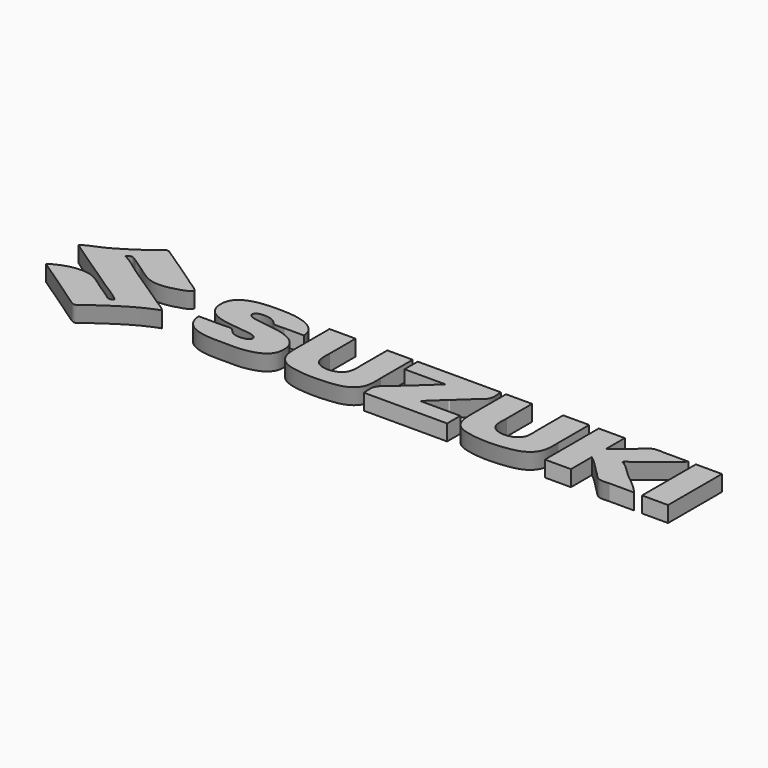
from build123d import *

# Parameters (mm, degrees)
F1_DEPTH = 25
F0_W     = 41
F0_H     = 106


# Not quite as in the source:
# - ends of sketch curves that miss each other by under 0.0002 mm in the source are joined


with BuildPart() as f1:
    # F0 (on Top) → F1 (new body)
    with BuildSketch(Plane.XY):
        Polygon((-498.7323, 35.60855), (-499.5, 35.04365), (-498.6864, 34.46155), (-497.8721, 33.88035), (-497.0571, 33.30005), (-496.2415, 32.72065), (-495.4252, 32.14205), (-494.6084, 31.56425), (-493.7909, 30.98735), (-492.9728, 30.41125), (-492.1542, 29.83595), (-491.335, 29.26135), (-490.5152, 28.68765), (-489.6948, 28.11455), (-488.874, 27.54235), (-488.0526, 26.97075), (-487.2306, 26.39985), (-486.4082, 25.82965), (-485.5852, 25.26015), (-484.7618, 24.69135), (-483.9379, 24.12315), (-483.1135, 23.55565), (-482.2887, 22.98865), (-481.4635, 22.42235), (-480.6378, 21.85655), (-479.8116, 21.29145), (-478.9851, 20.72675), (-478.1582, 20.16275), (-477.3309, 19.59915), (-476.5032, 19.03615), (-475.6751, 18.47365), (-474.8467, 17.91155), (-474.0179, 17.35005), (-473.1888, 16.78895), (-472.3594, 16.22825), (-471.5297, 15.66795), (-470.6997, 15.10815), (-469.8693, 14.54875), (-469.0387, 13.98965), (-468.2078, 13.43095), (-467.3767, 12.87265), (-466.5453, 12.31465), (-465.7137, 11.75695), (-464.8819, 11.19965), (-464.0498, 10.64255), (-463.2176, 10.08575), (-462.3851, 9.52925), (-461.5525, 8.97295), (-460.7197, 8.41695), (-459.8868, 7.86115), (-459.0537, 7.30555), (-458.2204, 6.75015), (-457.387, 6.19495), (-456.5536, 5.63985), (-455.72, 5.08495), (-454.8863, 4.53015), (-454.0525, 3.97545), (-453.2187, 3.42085), (-452.3848, 2.86635), (-451.5508, 2.31195), (-450.7168, 1.75765), (-449.8828, 1.20335), (-449.0488, 0.64905), (-448.2148, 0.09485), (-447.3807, -0.45945), (-446.5467, -1.01365), (-445.7127, -1.56795), (-444.8787, -2.12235), (-444.0448, -2.67665), (-443.211, -3.23115), (-442.3772, -3.78575), (-441.5435, -4.34035), (-440.7099, -4.89515), (-439.8764, -5.45005), (-439.043, -6.00505), (-438.2098, -6.56025), (-437.3766, -7.11565), (-436.5436, -7.67125), (-435.7108, -8.22695), (-434.8782, -8.78295), (-434.0457, -9.33915), (-433.2134, -9.89565), (-432.3813, -10.45245), (-431.5494, -11.00945), (-430.7178, -11.56675), (-429.8864, -12.12435), (-429.0552, -12.68225), (-428.2243, -13.24055), (-427.3936, -13.79915), (-426.5633, -14.35815), (-425.7332, -14.91745), (-424.9034, -15.47725), (-424.0739, -16.03745), (-423.2448, -16.59805), (-422.416, -17.15905), (-421.5875, -17.72055), (-420.7594, -18.28245), (-419.9316, -18.84495), (-419.1042, -19.40785), (-418.2772, -19.97135), (-417.4507, -20.53525), (-416.6245, -21.09975), (-415.7987, -21.66485), (-414.9734, -22.23055), (-414.1485, -22.79675), (-413.324, -23.36355), (-412.5, -23.93095), (-411.6765, -24.49535), (-410.8486, -25.05655), (-410.0166, -25.61485), (-409.1807, -26.17045), (-408.3413, -26.72355), (-407.4987, -27.27445), (-406.653, -27.82335), (-405.8047, -28.37065), (-404.9538, -28.91635), (-404.1008, -29.46085), (-403.2459, -30.00435), (-402.3893, -30.54705), (-401.5314, -31.08935), (-400.6724, -31.63125), (-399.8126, -32.17325), (-398.9522, -32.71535), (-398.0916, -33.25805), (-397.2309, -33.80135), (-396.3706, -34.34565), (-395.5108, -34.89105), (-394.6518, -35.43795), (-393.7939, -35.98655), (-392.9373, -36.53705), (-392.0824, -37.08975), (-391.2295, -37.64475), (-390.3787, -38.20245), (-389.5303, -38.76305), (-388.6847, -39.32685), (-387.8421, -39.89395), (-387.0028, -40.46465), (-386.167, -41.03925), (-385.3351, -41.61795), (-384.5072, -42.20105), (-383.6837, -42.78865), (-382.8649, -43.38115), (-382.0509, -43.97865), (-381.2422, -44.58155), (-380.4389, -45.19005), (-379.6413, -45.80425), (-378.8498, -46.42455), (-378.0645, -47.05115), (-377.2858, -47.68425), (-376.5139, -48.32415), (-375.7491, -48.97105), (-374.9917, -49.62525), (-374.2419, -50.28695), (-373.5, -50.95635), (-374.3581, -51.38155), (-375.2655, -51.86565), (-376.2089, -52.36255), (-377.175, -52.82615), (-378.1506, -53.21035), (-379.1225, -53.46895), (-380.0772, -53.55595), (-380.972, -53.46095), (-381.8777, -53.21815), (-382.7883, -52.85145), (-383.6974, -52.38435), (-384.5988, -51.84045), (-385.4865, -51.24355), (-386.3541, -50.61715), (-387.1955, -49.98495), (-388.0044, -49.37055), (-388.7746, -48.79765), (-389.5, -48.28975), (-409.5, -34.95635), (-410.3052, -34.41505), (-411.1114, -33.86445), (-411.9189, -33.30565), (-412.7278, -32.73955), (-413.5382, -32.16715), (-414.3504, -31.58965), (-415.1643, -31.00785), (-415.9802, -30.42275), (-416.7981, -29.83555), (-417.6183, -29.24705), (-418.4409, -28.65835), (-419.2659, -28.07045), (-420.0936, -27.48435), (-420.924, -26.90105), (-421.7574, -26.32155), (-422.5937, -25.74685), (-423.4333, -25.17805), (-424.2761, -24.61595), (-425.1225, -24.06175), (-425.9723, -23.51625), (-426.826, -22.98065), (-427.6834, -22.45595), (-428.5449, -21.94305), (-429.4105, -21.44295), (-430.2803, -20.95665), (-431.1545, -20.48535), (-432.0333, -20.02975), (-432.9168, -19.59115), (-433.805, -19.17025), (-434.6983, -18.76835), (-435.5965, -18.38625), (-436.5, -18.02505), (-437.4101, -17.68515), (-438.3275, -17.36615), (-439.252, -17.06775), (-440.1832, -16.78965), (-441.1208, -16.53165), (-442.0644, -16.29335), (-443.0137, -16.07465), (-443.9683, -15.87525), (-444.928, -15.69485), (-445.8923, -15.53315), (-446.8609, -15.38995), (-447.8336, -15.26485), (-448.8098, -15.15775), (-449.7894, -15.06825), (-450.7719, -14.99615), (-451.757, -14.94115), (-452.7445, -14.90295), (-453.7338, -14.88145), (-454.7247, -14.87615), (-455.7169, -14.88695), (-456.71, -14.91345), (-457.7037, -14.95555), (-458.6976, -15.01285), (-459.6914, -15.08505), (-460.6847, -15.17205), (-461.6772, -15.27335), (-462.6686, -15.38885), (-463.6585, -15.51825), (-464.6466, -15.66135), (-465.6325, -15.81775), (-466.6159, -15.98715), (-467.5965, -16.16945), (-468.5739, -16.36425), (-469.5478, -16.57135), (-470.5178, -16.79045), (-471.4835, -17.02125), (-472.4448, -17.26355), (-473.4011, -17.51705), (-474.3522, -17.78155), (-475.2977, -18.05665), (-476.2373, -18.34215), (-477.1706, -18.63775), (-478.0974, -18.94325), (-479.0172, -19.25825), (-479.9297, -19.58265), (-480.8346, -19.91605), (-481.7315, -20.25835), (-482.6201, -20.60905), (-483.5, -20.96795), (-484.4491, -21.36105), (-485.4051, -21.75885), (-486.3651, -22.16375), (-487.3259, -22.57815), (-488.2846, -23.00465), (-489.238, -23.44565), (-490.1831, -23.90365), (-491.1168, -24.38095), (-492.036, -24.88025), (-492.9377, -25.40375), (-493.8187, -25.95415), (-494.6761, -26.53375), (-495.5067, -27.14505), (-496.3074, -27.79045), (-497.0753, -28.47255), (-497.8072, -29.19375), (-498.5, -29.95635), (-497.6616, -30.52175), (-496.823, -31.08685), (-495.9841, -31.65165), (-495.145, -32.21625), (-494.3057, -32.78065), (-493.4661, -33.34475), (-492.6264, -33.90865), (-491.7865, -34.47245), (-490.9464, -35.03595), (-490.1061, -35.59935), (-489.2657, -36.16255), (-488.4251, -36.72555), (-487.5844, -37.28855), (-486.7436, -37.85135), (-485.9027, -38.41405), (-485.0617, -38.97665), (-484.2205, -39.53925), (-483.3793, -40.10165), (-482.5381, -40.66415), (-481.6967, -41.22645), (-480.8553, -41.78885), (-480.0139, -42.35115), (-479.1725, -42.91355), (-478.331, -43.47585), (-477.4895, -44.03825), (-476.648, -44.60065), (-475.8066, -45.16305), (-474.9651, -45.72555), (-474.1237, -46.28815), (-473.2823, -46.85085), (-472.441, -47.41355), (-471.5998, -47.97645), (-470.7586, -48.53945), (-469.9175, -49.10265), (-469.0765, -49.66595), (-468.2356, -50.22945), (-467.3949, -50.79305), (-466.5542, -51.35685), (-465.7137, -51.92095), (-464.8734, -52.48515), (-464.0332, -53.04965), (-463.1931, -53.61445), (-462.3533, -54.17935), (-461.5136, -54.74465), (-460.6742, -55.31015), (-459.8349, -55.87595), (-458.9959, -56.44215), (-458.1571, -57.00855), (-457.3185, -57.57535), (-456.4802, -58.14245), (-455.6422, -58.70995), (-454.8044, -59.27785), (-453.9669, -59.84605), (-453.1297, -60.41475), (-452.2929, -60.98375), (-451.4563, -61.55325), (-450.62, -62.12315), (-449.7841, -62.69345), (-448.9486, -63.26435), (-448.1134, -63.83555), (-447.2785, -64.40735), (-446.444, -64.97965), (-445.61, -65.55245), (-444.7763, -66.12575), (-443.943, -66.69965), (-443.1102, -67.27405), (-442.2777, -67.84895), (-441.4458, -68.42455), (-440.6142, -69.00065), (-439.7832, -69.57745), (-438.9525, -70.15475), (-438.1224, -70.73275), (-437.2928, -71.31135), (-436.4637, -71.89065), (-435.6351, -72.47055), (-434.807, -73.05125), (-433.9794, -73.63255), (-433.1524, -74.21455), (-432.3259, -74.79735), (-431.5, -75.38075), (-430.6526, -75.97855), (-429.8038, -76.57425), (-428.9538, -77.16785), (-428.1027, -77.75965), (-427.2503, -78.34955), (-426.3969, -78.93785), (-425.5424, -79.52445), (-424.687, -80.10955), (-423.8306, -80.69325), (-422.9733, -81.27565), (-422.1152, -81.85685), (-421.2563, -82.43695), (-420.3967, -83.01595), (-419.5365, -83.59405), (-418.6756, -84.17135), (-417.8141, -84.74785), (-416.9521, -85.32385), (-416.0897, -85.89915), (-415.2268, -86.47415), (-414.3636, -87.04875), (-413.5, -87.62305), (-412.7161, -88.16295), (-411.8976, -88.74755), (-411.048, -89.35185), (-410.1704, -89.95065), (-409.2681, -90.51895), (-408.3444, -91.03155), (-407.4025, -91.46355), (-406.4456, -91.78975), (-405.4771, -91.98495), (-404.5, -92.02425), (-403.5757, -91.90875), (-402.6608, -91.66295), (-401.7575, -91.30465), (-400.8679, -90.85175), (-399.9942, -90.32195), (-399.1385, -89.73305), (-398.3029, -89.10295), (-397.4894, -88.44935), (-396.7003, -87.79015), (-395.9376, -87.14305), (-395.2035, -86.52585), (-394.5, -85.95635), (-393.7037, -85.33445), (-392.9045, -84.71645), (-392.1026, -84.10225), (-391.2979, -83.49165), (-390.4908, -82.88455), (-389.6813, -82.28075), (-388.8695, -81.68005), (-388.0555, -81.08225), (-387.2394, -80.48735), (-386.4215, -79.89495), (-385.6017, -79.30515), (-384.7803, -78.71755), (-383.9573, -78.13215), (-383.1329, -77.54875), (-382.3071, -76.96715), (-381.4802, -76.38715), (-380.6522, -75.80865), (-379.8232, -75.23145), (-378.9934, -74.65535), (-378.1628, -74.08035), (-377.3317, -73.50605), (-376.5, -72.93245), (-375.6869, -72.37275), (-374.8717, -71.81305), (-374.0545, -71.25345), (-373.2353, -70.69405), (-372.4141, -70.13495), (-371.591, -69.57625), (-370.7658, -69.01805), (-369.9387, -68.46045), (-369.1096, -67.90345), (-368.2786, -67.34715), (-367.4456, -66.79175), (-366.6107, -66.23725), (-365.7739, -65.68375), (-364.9351, -65.13135), (-364.0945, -64.58015), (-363.2519, -64.03015), (-362.4075, -63.48155), (-361.5612, -62.93435), (-360.713, -62.38875), (-359.863, -61.84465), (-359.0111, -61.30235), (-358.1573, -60.76175), (-357.3017, -60.22315), (-356.4443, -59.68635), (-355.5851, -59.15175), (-354.7241, -58.61915), (-353.8612, -58.08885), (-352.9966, -57.56085), (-352.1302, -57.03525), (-351.262, -56.51215), (-350.3921, -55.99155), (-349.5204, -55.47365), (-348.6469, -54.95855), (-347.7717, -54.44625), (-346.8948, -53.93685), (-346.0162, -53.43045), (-345.1358, -52.92715), (-344.2537, -52.42705), (-343.37, -51.93025), (-342.4845, -51.43675), (-341.5974, -50.94665), (-340.7086, -50.46015), (-339.8182, -49.97725), (-338.9261, -49.49815), (-338.0324, -49.02275), (-337.137, -48.55115), (-336.24, -48.08365), (-335.3414, -47.62015), (-334.4411, -47.16075), (-333.5393, -46.70565), (-332.6359, -46.25485), (-331.7309, -45.80845), (-330.8244, -45.36645), (-329.9162, -44.92915), (-329.0065, -44.49645), (-328.0953, -44.06855), (-327.1826, -43.64545), (-326.2683, -43.22725), (-325.3525, -42.81415), (-324.4351, -42.40605), (-323.5163, -42.00315), (-322.596, -41.60555), (-321.6742, -41.21335), (-320.7509, -40.82655), (-319.8262, -40.44535), (-318.9, -40.06965), (-317.9723, -39.69975), (-317.0432, -39.33565), (-316.1127, -38.97735), (-315.1808, -38.62515), (-314.2474, -38.27895), (-313.3127, -37.93885), (-312.3765, -37.60505), (-311.439, -37.27755), (-310.5, -36.95635), (-311.1437, -36.21015), (-311.8162, -35.49105), (-312.5153, -34.79735), (-313.2387, -34.12695), (-313.9843, -33.47825), (-314.7499, -32.84925), (-315.5331, -32.23805), (-316.3317, -31.64295), (-317.1437, -31.06205), (-317.9666, -30.49335), (-318.7982, -29.93515), (-319.6365, -29.38555), (-320.479, -28.84275), (-321.3236, -28.30475), (-322.1681, -27.76975), (-323.0102, -27.23595), (-323.8478, -26.70155), (-324.6784, -26.16455), (-325.5, -25.62305), (-353.5, -6.95635), (-354.3422, -6.39525), (-355.1847, -5.83445), (-356.0274, -5.27405), (-356.8705, -4.71405), (-357.7137, -4.15425), (-358.5572, -3.59475), (-359.401, -3.03555), (-360.2449, -2.47665), (-361.089, -1.91795), (-361.9333, -1.35935), (-362.7777, -0.80105), (-363.6223, -0.24285), (-364.467, 0.31515), (-365.3118, 0.87315), (-366.1567, 1.43095), (-367.0017, 1.98875), (-367.8467, 2.54645), (-368.6917, 3.10415), (-369.5368, 3.66185), (-370.3818, 4.21955), (-371.2269, 4.77735), (-372.0719, 5.33515), (-372.9169, 5.89305), (-373.7618, 6.45105), (-374.6066, 7.00925), (-375.4514, 7.56745), (-376.296, 8.12595), (-377.1405, 8.68465), (-377.9848, 9.24345), (-378.829, 9.80255), (-379.673, 10.36195), (-380.5168, 10.92155), (-381.3604, 11.48155), (-382.2038, 12.04185), (-383.0469, 12.60245), (-383.8898, 13.16345), (-384.7324, 13.72485), (-385.5747, 14.28665), (-386.4167, 14.84885), (-387.2583, 15.41155), (-388.0996, 15.97475), (-388.9405, 16.53845), (-389.7811, 17.10265), (-390.6213, 17.66745), (-391.461, 18.23275), (-392.3004, 18.79865), (-393.1393, 19.36515), (-393.9777, 19.93235), (-394.8156, 20.50015), (-395.6531, 21.06865), (-396.49, 21.63785), (-397.3265, 22.20775), (-398.1623, 22.77845), (-398.9976, 23.34985), (-399.8324, 23.92215), (-400.6665, 24.49515), (-401.5, 25.06905), (-402.3053, 25.62655), (-403.1108, 26.18905), (-403.9167, 26.75605), (-404.7231, 27.32715), (-405.53, 27.90195), (-406.3374, 28.48015), (-407.1456, 29.06115), (-407.9546, 29.64465), (-408.7644, 30.23025), (-409.5752, 30.81755), (-410.3869, 31.40605), (-411.1998, 31.99545), (-412.0138, 32.58525), (-412.8291, 33.17515), (-413.6458, 33.76455), (-414.4639, 34.35325), (-415.2835, 34.94075), (-416.1046, 35.52665), (-416.9275, 36.11055), (-417.7521, 36.69195), (-418.5785, 37.27065), (-419.4068, 37.84595), (-420.2371, 38.41775), (-421.0695, 38.98535), (-421.9041, 39.54865), (-422.7409, 40.10695), (-423.58, 40.65995), (-424.4215, 41.20735), (-425.2655, 41.74865), (-426.112, 42.28335), (-426.9612, 42.81115), (-427.8131, 43.33165), (-428.6679, 43.84445), (-429.5255, 44.34905), (-430.3861, 44.84515), (-431.2497, 45.33225), (-432.1164, 45.80995), (-432.9864, 46.27785), (-433.8597, 46.73565), (-434.7363, 47.18275), (-435.6164, 47.61885), (-436.5, 48.04365), (-435.7159, 48.58385), (-434.9012, 49.15915), (-434.0578, 49.74165), (-433.1876, 50.30355), (-432.2925, 50.81705), (-431.3743, 51.25445), (-430.4349, 51.58785), (-429.4762, 51.78945), (-428.5, 51.83145), (-427.5328, 51.70405), (-426.5801, 51.43285), (-425.6441, 51.04405), (-424.7269, 50.56375), (-423.8308, 50.01835), (-422.9579, 49.43405), (-422.1103, 48.83705), (-421.2903, 48.25375), (-420.5, 47.71025), (-404.5, 37.04365), (-403.698, 36.50495), (-402.8948, 35.95805), (-402.0902, 35.40375), (-401.2843, 34.84265), (-400.4768, 34.27555), (-399.6677, 33.70325), (-398.8569, 33.12635), (-398.0443, 32.54575), (-397.2298, 31.96205), (-396.4133, 31.37605), (-395.5947, 30.78855), (-394.7739, 30.20025), (-393.9508, 29.61185), (-393.1253, 29.02415), (-392.2973, 28.43775), (-391.4667, 27.85365), (-390.6334, 27.27235), (-389.7973, 26.69465), (-388.9584, 26.12135), (-388.1164, 25.55325), (-387.2714, 24.99085), (-386.4232, 24.43515), (-385.5717, 23.88675), (-384.7169, 23.34635), (-383.8586, 22.81485), (-382.9967, 22.29295), (-382.1311, 21.78125), (-381.2618, 21.28055), (-380.3886, 20.79175), (-379.5114, 20.31535), (-378.6302, 19.85225), (-377.7448, 19.40315), (-376.8551, 18.96885), (-375.9611, 18.54995), (-375.0626, 18.14725), (-374.1596, 17.76155), (-373.252, 17.39355), (-372.3395, 17.04395), (-371.4223, 16.71355), (-370.5, 16.40315), (-369.6067, 16.12685), (-368.6997, 15.87325), (-367.7797, 15.64185), (-366.8476, 15.43225), (-365.9041, 15.24405), (-364.95, 15.07675), (-363.986, 14.92995), (-363.0129, 14.80315), (-362.0314, 14.69585), (-361.0424, 14.60775), (-360.0466, 14.53845), (-359.0447, 14.48725), (-358.0376, 14.45395), (-357.0259, 14.43795), (-356.0104, 14.43895), (-354.992, 14.45635), (-353.9714, 14.48985), (-352.9493, 14.53895), (-351.9265, 14.60315), (-350.9037, 14.68215), (-349.8818, 14.77535), (-348.8615, 14.88235), (-347.8435, 15.00275), (-346.8287, 15.13615), (-345.8177, 15.28195), (-344.8114, 15.43985), (-343.8105, 15.60935), (-342.8158, 15.79005), (-341.828, 15.98145), (-340.8479, 16.18315), (-339.8763, 16.39465), (-338.914, 16.61555), (-337.9616, 16.84535), (-337.02, 17.08375), (-336.0899, 17.33015), (-335.1721, 17.58425), (-334.2673, 17.84545), (-333.3764, 18.11345), (-332.5, 18.38775), (-331.7359, 18.62475), (-330.9132, 18.86935), (-330.0393, 19.12285), (-329.1212, 19.38655), (-328.1662, 19.66175), (-327.1814, 19.94995), (-326.1742, 20.25235), (-325.1515, 20.57035), (-324.1208, 20.90545), (-323.0891, 21.25875), (-322.0636, 21.63175), (-321.0515, 22.02585), (-320.0601, 22.44225), (-319.0964, 22.88235), (-318.1678, 23.34755), (-317.2814, 23.83915), (-316.4443, 24.35855), (-315.6638, 24.90705), (-314.9472, 25.48605), (-314.3014, 26.09685), (-313.7339, 26.74085), (-313.2516, 27.41945), (-312.846, 28.30935), (-312.7444, 29.15205), (-312.8988, 29.94715), (-313.2614, 30.69415), (-313.7843, 31.39275), (-314.4195, 32.04255), (-315.1191, 32.64325), (-315.8353, 33.19435), (-316.5201, 33.69565), (-317.342, 34.28855), (-318.1693, 34.87405), (-319.0016, 35.45295), (-319.8381, 36.02595), (-320.6783, 36.59405), (-321.5216, 37.15775), (-322.3675, 37.71815), (-323.2153, 38.27595), (-324.0644, 38.83185), (-324.9143, 39.38675), (-325.7644, 39.94145), (-326.614, 40.49675), (-327.4627, 41.05345), (-328.3097, 41.61235), (-329.1545, 42.17425), (-329.9965, 42.73995), (-330.8352, 43.31025), (-331.6699, 43.88595), (-332.5, 44.46795), (-333.324, 45.04995), (-334.1486, 45.63125), (-334.974, 46.21175), (-335.8, 46.79145), (-336.6266, 47.37045), (-337.4539, 47.94885), (-338.2818, 48.52645), (-339.1103, 49.10335), (-339.9394, 49.67955), (-340.7691, 50.25515), (-341.5994, 50.83005), (-342.4302, 51.40435), (-343.2615, 51.97795), (-344.0934, 52.55105), (-344.9257, 53.12345), (-345.7586, 53.69535), (-346.5919, 54.26665), (-347.4257, 54.83735), (-348.2599, 55.40755), (-349.0945, 55.97715), (-349.9296, 56.54635), (-350.7651, 57.11495), (-351.6009, 57.68315), (-352.4371, 58.25085), (-353.2737, 58.81805), (-354.1106, 59.38475), (-354.9478, 59.95115), (-355.7854, 60.51705), (-356.6232, 61.08255), (-357.4613, 61.64765), (-358.2997, 62.21235), (-359.1384, 62.77675), (-359.9772, 63.34075), (-360.8163, 63.90435), (-361.6556, 64.46775), (-362.4951, 65.03075), (-363.3347, 65.59345), (-364.1745, 66.15585), (-365.0145, 66.71805), (-365.8546, 67.27995), (-366.6948, 67.84155), (-367.5351, 68.40305), (-368.3755, 68.96425), (-369.216, 69.52515), (-370.0565, 70.08595), (-370.897, 70.64665), (-371.7376, 71.20705), (-372.5782, 71.76735), (-373.4188, 72.32755), (-374.2594, 72.88755), (-375.0999, 73.44755), (-375.9404, 74.00735), (-376.7808, 74.56705), (-377.6211, 75.12675), (-378.4614, 75.68635), (-379.3015, 76.24595), (-380.1415, 76.80545), (-380.9814, 77.36495), (-381.8211, 77.92455), (-382.6607, 78.48405), (-383.5, 79.04365), (-397.5, 88.376231), (-398.2831, 88.91135), (-399.0983, 89.48445), (-399.9427, 90.06515), (-400.8133, 90.62315), (-401.7074, 91.12835), (-402.6218, 91.55035), (-403.5536, 91.85915), (-404.5, 92.02435), (-405.5277, 92.00595), (-406.5196, 91.79065), (-407.476, 91.41245), (-408.3976, 90.90535), (-409.2848, 90.30355), (-410.1382, 89.64095), (-410.9582, 88.95165), (-411.7453, 88.26975), (-412.5, 87.62925), (-413.2855, 86.98145), (-414.0703, 86.33315), (-414.8547, 85.68465), (-415.6392, 85.03655), (-416.4241, 84.38915), (-417.2099, 83.74305), (-417.9968, 83.09845), (-418.7852, 82.45605), (-419.5755, 81.81615), (-420.3681, 81.17915), (-421.1633, 80.54555), (-421.9616, 79.91585), (-422.7632, 79.29045), (-423.5685, 78.66965), (-424.378, 78.05415), (-425.192, 77.44415), (-426.0108, 76.84015), (-426.8348, 76.24275), (-427.6645, 75.65215), (-428.5, 75.06905), (-429.3259, 74.49915), (-430.1527, 73.92995), (-430.9805, 73.36155), (-431.8093, 72.79385), (-432.6392, 72.22695), (-433.4702, 71.66105), (-434.3022, 71.09625), (-435.1354, 70.53245), (-435.9697, 69.96975), (-436.8051, 69.40835), (-437.6418, 68.84835), (-438.4796, 68.28965), (-439.3186, 67.73245), (-440.1589, 67.17675), (-441.0004, 66.62275), (-441.8431, 66.07035), (-442.6872, 65.51985), (-443.5326, 64.97105), (-444.3793, 64.42425), (-445.2274, 63.87945), (-446.0768, 63.33675), (-446.9277, 62.79615), (-447.7799, 62.25785), (-448.6336, 61.72175), (-449.4888, 61.18815), (-450.3454, 60.65695), (-451.2035, 60.12825), (-452.0631, 59.60215), (-452.9242, 59.07875), (-453.7869, 58.55815), (-454.6512, 58.04035), (-455.5171, 57.52545), (-456.3845, 57.01355), (-457.2537, 56.50475), (-458.1244, 55.99905), (-458.9969, 55.49655), (-459.871, 54.99735), (-460.7469, 54.50155), (-461.6244, 54.00915), (-462.5038, 53.52025), (-463.3849, 53.03495), (-464.2678, 52.55335), (-465.1525, 52.07555), (-466.0391, 51.60145), (-466.9275, 51.13135), (-467.8178, 50.66515), (-468.7099, 50.20305), (-469.604, 49.74505), (-470.5, 49.29125), (-471.3645, 48.86275), (-472.2433, 48.43985), (-473.1352, 48.02185), (-474.0391, 47.60805), (-474.9539, 47.19785), (-475.8784, 46.79055), (-476.8113, 46.38545), (-477.7516, 45.98205), (-478.6981, 45.57945), (-479.6497, 45.17705), (-480.6051, 44.77435), (-481.5631, 44.37055), (-482.5228, 43.96495), (-483.4828, 43.55695), (-484.442, 43.14595), (-485.3992, 42.73115), (-486.3533, 42.31185), (-487.3032, 41.88765), (-488.2476, 41.45765), (-489.1854, 41.02125), (-490.1154, 40.57775), (-491.0365, 40.12655), (-491.9475, 39.66695), (-492.8472, 39.19835), (-493.7345, 38.71995), (-494.6082, 38.23125), (-495.4672, 37.73145), (-496.3102, 37.21995), (-497.1362, 36.69615), (-497.9439, 36.15925), align=None)
    extrude(amount=F1_DEPTH)


with BuildPart() as f1b:
    # F0 (on Top) → F1, piece 2 (new body)
    with BuildSketch(Plane.XY):
        Polygon((-229.5, -20.95635), (-265.5, -20.95635), (-265.3637, -21.97995), (-265.2167, -23.00855), (-265.0573, -24.04065), (-264.8834, -25.07425), (-264.6932, -26.10775), (-264.4847, -27.13925), (-264.2559, -28.16705), (-264.005, -29.18935), (-263.73, -30.20445), (-263.4289, -31.21035), (-263.0999, -32.20545), (-262.741, -33.18805), (-262.3503, -34.15615), (-261.9257, -35.10805), (-261.4655, -36.04215), (-260.9676, -36.95635), (-260.49, -37.76275), (-259.9928, -38.54735), (-259.4767, -39.31035), (-258.9419, -40.05215), (-258.3888, -40.77305), (-257.8179, -41.47335), (-257.2295, -42.15325), (-256.624, -42.81315), (-256.0018, -43.45325), (-255.3633, -44.07395), (-254.7089, -44.67555), (-254.0389, -45.25825), (-253.3539, -45.82235), (-252.6541, -46.36825), (-251.94, -46.89625), (-251.2119, -47.40655), (-250.4702, -47.89945), (-249.7154, -48.37535), (-248.9478, -48.83445), (-248.1678, -49.27705), (-247.3759, -49.70355), (-246.5723, -50.11415), (-245.7575, -50.50925), (-244.9318, -50.88895), (-244.0958, -51.25375), (-243.2497, -51.60385), (-242.3939, -51.93955), (-241.5289, -52.26115), (-240.6551, -52.56905), (-239.7727, -52.86335), (-238.8823, -53.14455), (-237.9842, -53.41275), (-237.0788, -53.66845), (-236.1664, -53.91185), (-235.2476, -54.14315), (-234.3226, -54.36285), (-233.3919, -54.57105), (-232.4559, -54.76825), (-231.5148, -54.95455), (-230.5693, -55.13035), (-229.6196, -55.29595), (-228.666, -55.45165), (-227.7092, -55.59765), (-226.7493, -55.73435), (-225.7868, -55.86205), (-224.8221, -55.98105), (-223.8555, -56.09155), (-222.8876, -56.19395), (-221.9186, -56.28855), (-220.9489, -56.37555), (-219.979, -56.45535), (-219.0093, -56.52825), (-218.04, -56.59435), (-217.0717, -56.65425), (-216.1047, -56.70805), (-215.1394, -56.75605), (-214.1762, -56.79865), (-213.2155, -56.83605), (-212.2576, -56.86865), (-211.303, -56.89665), (-210.3521, -56.92035), (-209.4052, -56.94015), (-208.4628, -56.95625), (-207.5252, -56.96895), (-206.5928, -56.97855), (-205.666, -56.98545), (-204.7453, -56.98985), (-203.8309, -56.99205), (-202.9233, -56.99235), (-202.0229, -56.99105), (-201.1301, -56.98845), (-200.2453, -56.98495), (-199.3688, -56.98065), (-198.501, -56.97605), (-197.6424, -56.97125), (-196.7933, -56.96675), (-195.9541, -56.96265), (-195.1253, -56.95935), (-194.3071, -56.95715), (-193.5, -56.95635), (-192.5014, -56.95845), (-191.5017, -56.96415), (-190.5012, -56.97275), (-189.5, -56.98345), (-188.4981, -56.99545), (-187.4956, -57.00815), (-186.4928, -57.02065), (-185.4896, -57.03225), (-184.4862, -57.04215), (-183.4827, -57.04975), (-182.4792, -57.05415), (-181.4758, -57.05455), (-180.4726, -57.05035), (-179.4697, -57.04075), (-178.4673, -57.02495), (-177.4654, -57.00215), (-176.4642, -56.97175), (-175.4637, -56.93285), (-174.4641, -56.88475), (-173.4655, -56.82675), (-172.4679, -56.75805), (-171.4715, -56.67785), (-170.4765, -56.58535), (-169.4828, -56.48005), (-168.4906, -56.36085), (-167.5, -56.22725), (-166.6409, -56.10265), (-165.7726, -55.97185), (-164.896, -55.83465), (-164.0119, -55.69065), (-163.1211, -55.53935), (-162.2245, -55.38035), (-161.3229, -55.21335), (-160.4172, -55.03785), (-159.5082, -54.85355), (-158.5967, -54.65995), (-157.6836, -54.45675), (-156.7698, -54.24355), (-155.856, -54.01985), (-154.9431, -53.78535), (-154.032, -53.53965), (-153.1234, -53.28225), (-152.2183, -53.01285), (-151.3175, -52.73105), (-150.4218, -52.43645), (-149.532, -52.12855), (-148.6491, -51.80705), (-147.7737, -51.47155), (-146.9069, -51.12165), (-146.0493, -50.75695), (-145.2019, -50.37705), (-144.3656, -49.98145), (-143.541, -49.56995), (-142.7291, -49.14205), (-141.9308, -48.69725), (-141.1468, -48.23535), (-140.378, -47.75585), (-139.6253, -47.25835), (-138.8894, -46.74245), (-138.1713, -46.20775), (-137.4717, -45.65385), (-136.7916, -45.08035), (-136.1317, -44.48695), (-135.4929, -43.87315), (-134.876, -43.23855), (-134.2818, -42.58275), (-133.7113, -41.90545), (-133.1652, -41.20615), (-132.6445, -40.48445), (-132.1498, -39.74005), (-131.6822, -38.97245), (-131.2423, -38.18135), (-130.8311, -37.36625), (-130.4494, -36.52675), (-130.098, -35.66255), (-129.7778, -34.77325), (-129.4897, -33.85835), (-129.2343, -32.91755), (-129.0127, -31.95035), (-128.8256, -30.95635), (-128.6801, -29.99165), (-128.5634, -29.00915), (-128.4738, -28.01225), (-128.4096, -27.00435), (-128.3689, -25.98905), (-128.35, -24.96945), (-128.3511, -23.94925), (-128.3703, -22.93165), (-128.406, -21.92015), (-128.4562, -20.91825), (-128.5193, -19.92915), (-128.5934, -18.95635), (-128.698, -17.96405), (-128.8467, -16.98705), (-129.0382, -16.02565), (-129.2711, -15.07995), (-129.5442, -14.15025), (-129.8561, -13.23685), (-130.2054, -12.33975), (-130.5908, -11.45945), (-131.011, -10.59585), (-131.4647, -9.74945), (-131.9504, -8.92025), (-132.4669, -8.10855), (-133.0129, -7.31465), (-133.5869, -6.53865), (-134.1877, -5.78075), (-134.8139, -5.04125), (-135.4641, -4.32035), (-136.1371, -3.61825), (-136.8315, -2.93525), (-137.546, -2.27135), (-138.2792, -1.62695), (-139.0298, -1.00225), (-139.7964, -0.39735), (-140.5778, 0.18745), (-141.3725, 0.75185), (-142.1793, 1.29575), (-142.9968, 1.81895), (-143.8236, 2.32115), (-144.6585, 2.80225), (-145.5, 3.26195), (-146.3942, 3.72765), (-147.2927, 4.17715), (-148.1956, 4.61065), (-149.1028, 5.02865), (-150.014, 5.43155), (-150.9293, 5.81975), (-151.8484, 6.19375), (-152.7713, 6.55385), (-153.6979, 6.90045), (-154.628, 7.23395), (-155.5615, 7.55495), (-156.4984, 7.86365), (-157.4385, 8.16055), (-158.3818, 8.44615), (-159.328, 8.72065), (-160.277, 8.98465), (-161.2289, 9.23845), (-162.1834, 9.48245), (-163.1405, 9.71725), (-164.1, 9.94305), (-165.0618, 10.16035), (-166.0258, 10.36955), (-166.9919, 10.57105), (-167.96, 10.76525), (-168.93, 10.95265), (-169.9018, 11.13355), (-170.8752, 11.30845), (-171.8501, 11.47765), (-172.8265, 11.64165), (-173.8042, 11.80095), (-174.7831, 11.95575), (-175.7631, 12.10665), (-176.744, 12.25395), (-177.7258, 12.39805), (-178.7084, 12.53945), (-179.6917, 12.67845), (-180.6754, 12.81565), (-181.6596, 12.95125), (-182.6441, 13.08575), (-183.6288, 13.21965), (-184.6136, 13.35325), (-185.5983, 13.48695), (-186.583, 13.62115), (-187.5673, 13.75645), (-188.5513, 13.89305), (-189.5349, 14.03145), (-190.5178, 14.17195), (-191.5, 14.31525), (-192.4558, 14.45025), (-193.4325, 14.57845), (-194.4273, 14.70205), (-195.4378, 14.82325), (-196.4613, 14.94415), (-197.4952, 15.06695), (-198.5369, 15.19385), (-199.5838, 15.32705), (-200.6334, 15.46865), (-201.6829, 15.62075), (-202.7299, 15.78575), (-203.7717, 15.96565), (-204.8056, 16.16265), (-205.8292, 16.37885), (-206.8398, 16.61665), (-207.8348, 16.87795), (-208.8116, 17.16515), (-209.7676, 17.48025), (-210.7001, 17.82555), (-211.6067, 18.20315), (-212.4846, 18.61535), (-213.2286, 19.01935), (-213.9691, 19.49135), (-214.6854, 20.02625), (-215.3571, 20.61885), (-215.9635, 21.26385), (-216.484, 21.95625), (-216.898, 22.69095), (-217.1848, 23.46255), (-217.324, 24.26605), (-217.2948, 25.09615), (-217.0767, 25.94785), (-216.649, 26.81595), (-216.1701, 27.48825), (-215.6073, 28.09655), (-214.9675, 28.64335), (-214.2572, 29.13135), (-213.483, 29.56315), (-212.6518, 29.94125), (-211.77, 30.26825), (-210.8444, 30.54685), (-209.8815, 30.77955), (-208.8882, 30.96885), (-207.8709, 31.11755), (-206.8364, 31.22815), (-205.7914, 31.30315), (-204.7424, 31.34525), (-203.6961, 31.35705), (-202.6592, 31.34115), (-201.6384, 31.30005), (-200.6402, 31.23635), (-199.6713, 31.15275), (-198.7385, 31.05175), (-197.8483, 30.93595), (-197.0074, 30.80795), (-196.2224, 30.67035), (-195.5, 30.52585), (-194.5073, 30.29465), (-193.5273, 30.02735), (-192.5616, 29.72295), (-191.6119, 29.38025), (-190.6795, 28.99825), (-189.7662, 28.57605), (-188.8735, 28.11245), (-188.0028, 27.60645), (-187.1559, 27.05705), (-186.3343, 26.46315), (-185.5394, 25.82375), (-184.7894, 25.14915), (-184.0633, 24.44155), (-183.3464, 23.72225), (-182.6239, 23.01265), (-181.8811, 22.33425), (-181.1031, 21.70855), (-180.2752, 21.15685), (-179.3826, 20.70065), (-178.4105, 20.36155), (-177.4915, 20.14565), (-176.5439, 19.98085), (-175.5719, 19.86165), (-174.5797, 19.78275), (-173.5713, 19.73885), (-172.5508, 19.72445), (-171.5224, 19.73435), (-170.4901, 19.76315), (-169.458, 19.80545), (-168.4302, 19.85585), (-167.4109, 19.90915), (-166.4041, 19.95995), (-165.414, 20.00285), (-164.4446, 20.03255), (-163.5, 20.04365), (-132.5, 20.04365), (-132.5393, 21.08375), (-132.6118, 22.10415), (-132.717, 23.10505), (-132.8542, 24.08655), (-133.0229, 25.04895), (-133.2225, 25.99235), (-133.4522, 26.91675), (-133.7116, 27.82255), (-133.9999, 28.70985), (-134.3166, 29.57875), (-134.6611, 30.42935), (-135.0327, 31.26205), (-135.4309, 32.07685), (-135.8549, 32.87385), (-136.3043, 33.65345), (-136.7783, 34.41555), (-137.2765, 35.16055), (-137.798, 35.88845), (-138.3424, 36.59945), (-138.9091, 37.29365), (-139.4973, 37.97145), (-140.1066, 38.63275), (-140.7362, 39.27785), (-141.3856, 39.90695), (-142.0541, 40.52005), (-142.7412, 41.11755), (-143.4462, 41.69935), (-144.1685, 42.26585), (-144.9075, 42.81705), (-145.6626, 43.35325), (-146.4331, 43.87445), (-147.2185, 44.38095), (-148.0182, 44.87285), (-148.8314, 45.35035), (-149.6576, 45.81365), (-150.4963, 46.26275), (-151.3467, 46.69805), (-152.2083, 47.11955), (-153.0804, 47.52745), (-153.9624, 47.92195), (-154.8538, 48.30315), (-155.7538, 48.67125), (-156.662, 49.02645), (-157.5776, 49.36885), (-158.5, 49.69875), (-159.4823, 50.03465), (-160.4649, 50.35655), (-161.448, 50.66455), (-162.4314, 50.95885), (-163.4154, 51.23985), (-164.3998, 51.50795), (-165.3848, 51.76325), (-166.3704, 52.00625), (-167.3567, 52.23705), (-168.3436, 52.45605), (-169.3312, 52.66365), (-170.3195, 52.85995), (-171.3086, 53.04545), (-172.2985, 53.22035), (-173.2893, 53.38495), (-174.281, 53.53955), (-175.2736, 53.68445), (-176.2672, 53.81995), (-177.2617, 53.94645), (-178.2574, 54.06415), (-179.254, 54.17335), (-180.2519, 54.27435), (-181.2508, 54.36755), (-182.251, 54.45315), (-183.2523, 54.53145), (-184.255, 54.60285), (-185.2589, 54.66755), (-186.2642, 54.72585), (-187.2709, 54.77815), (-188.279, 54.82465), (-189.2885, 54.86575), (-190.2995, 54.90165), (-191.3121, 54.93265), (-192.3262, 54.95915), (-193.3419, 54.98145), (-194.3593, 54.99975), (-195.3783, 55.01435), (-196.3991, 55.02575), (-197.4216, 55.03395), (-198.4459, 55.03955), (-199.4721, 55.04265), (-200.5, 55.04365), (-201.5145, 55.04315), (-202.5274, 55.04155), (-203.5389, 55.03845), (-204.5489, 55.03355), (-205.5577, 55.02625), (-206.5652, 55.01645), (-207.5715, 55.00355), (-208.5766, 54.98735), (-209.5807, 54.96735), (-210.5837, 54.94315), (-211.5857, 54.91455), (-212.5868, 54.88115), (-213.5871, 54.84235), (-214.5865, 54.79805), (-215.5852, 54.74775), (-216.5832, 54.69105), (-217.5806, 54.62755), (-218.5774, 54.55705), (-219.5737, 54.47905), (-220.5695, 54.39315), (-221.565, 54.29905), (-222.56, 54.19635), (-223.5549, 54.08475), (-224.5494, 53.96365), (-225.5439, 53.83295), (-226.5382, 53.69215), (-227.5324, 53.54085), (-228.5267, 53.37865), (-229.521, 53.20535), (-230.5154, 53.02035), (-231.51, 52.82345), (-232.5049, 52.61425), (-233.5, 52.39235), (-234.4364, 52.17305), (-235.3773, 51.94355), (-236.3216, 51.70305), (-237.2682, 51.45105), (-238.216, 51.18685), (-239.1639, 50.90985), (-240.1108, 50.61945), (-241.0557, 50.31505), (-241.9974, 49.99605), (-242.9349, 49.66185), (-243.867, 49.31175), (-244.7927, 48.94515), (-245.7108, 48.56145), (-246.6203, 48.16005), (-247.5201, 47.74035), (-248.409, 47.30165), (-249.286, 46.84335), (-250.1501, 46.36495), (-251, 45.86575), (-251.8347, 45.34515), (-252.6531, 44.80255), (-253.4541, 44.23725), (-254.2366, 43.64865), (-254.9995, 43.03625), (-255.7418, 42.39935), (-256.4623, 41.73725), (-257.1599, 41.04955), (-257.8336, 40.33545), (-258.4822, 39.59435), (-259.1047, 38.82575), (-259.6999, 38.02895), (-260.2651, 37.20315), (-260.7937, 36.35545), (-261.286, 35.48725), (-261.7423, 34.60025), (-262.1627, 33.69585), (-262.5474, 32.77565), (-262.8968, 31.84115), (-263.211, 30.89395), (-263.4902, 29.93565), (-263.7348, 28.96765), (-263.9448, 27.99155), (-264.1206, 27.00885), (-264.2623, 26.02125), (-264.3702, 25.03005), (-264.4445, 24.03705), (-264.4854, 23.04365), (-264.5024, 22.02775), (-264.5019, 21.01505), (-264.4816, 20.00555), (-264.4393, 18.99935), (-264.3725, 17.99625), (-264.279, 16.99625), (-264.1564, 15.99955), (-264.0025, 15.00585), (-263.815, 14.01535), (-263.5914, 13.02795), (-263.3295, 12.04365), (-263.05, 11.12245), (-262.7466, 10.22465), (-262.4197, 9.34985), (-262.0699, 8.49765), (-261.6976, 7.66785), (-261.3033, 6.86005), (-260.8873, 6.07395), (-260.4501, 5.30905), (-259.9922, 4.56525), (-259.514, 3.84205), (-259.0159, 3.13925), (-258.4985, 2.45635), (-257.9622, 1.79315), (-257.4073, 1.14925), (-256.8344, 0.52435), (-256.2439, -0.08185), (-255.6362, -0.66975), (-255.0118, -1.23975), (-254.3712, -1.79205), (-253.7147, -2.32705), (-253.0429, -2.84515), (-252.3562, -3.34645), (-251.6549, -3.83155), (-250.9397, -4.30065), (-250.2108, -4.75415), (-249.4689, -5.19235), (-248.7142, -5.61555), (-247.9473, -6.02415), (-247.1686, -6.41845), (-246.3785, -6.79875), (-245.5776, -7.16545), (-244.7661, -7.51885), (-243.9447, -7.85935), (-243.1137, -8.18715), (-242.2736, -8.50275), (-241.4249, -8.80625), (-240.5679, -9.09825), (-239.7031, -9.37895), (-238.831, -9.64875), (-237.952, -9.90785), (-237.0666, -10.15675), (-236.1752, -10.39565), (-235.2782, -10.62495), (-234.3762, -10.84505), (-233.4695, -11.05615), (-232.5586, -11.25865), (-231.6439, -11.45285), (-230.726, -11.63915), (-229.8051, -11.81785), (-228.8819, -11.98935), (-227.9567, -12.15385), (-227.0299, -12.31175), (-226.1021, -12.46345), (-225.1737, -12.60915), (-224.2451, -12.74925), (-223.3167, -12.88415), (-222.389, -13.01415), (-221.4625, -13.13955), (-220.5377, -13.26075), (-219.6148, -13.37795), (-218.6945, -13.49165), (-217.7771, -13.60205), (-216.8631, -13.70955), (-215.9529, -13.81445), (-215.047, -13.91715), (-214.1459, -14.01795), (-213.2499, -14.11715), (-212.3596, -14.21515), (-211.4753, -14.31225), (-210.5975, -14.40875), (-209.7267, -14.50505), (-208.8633, -14.60135), (-208.0078, -14.69825), (-207.1606, -14.79585), (-206.3221, -14.89455), (-205.4928, -14.99475), (-204.6732, -15.09665), (-203.8637, -15.20075), (-203.0647, -15.30725), (-202.2766, -15.41645), (-201.5, -15.52885), (-200.5897, -15.65515), (-199.656, -15.76975), (-198.7016, -15.87565), (-197.7294, -15.97595), (-196.7421, -16.07335), (-195.7427, -16.17095), (-194.7339, -16.27145), (-193.7185, -16.37795), (-192.6994, -16.49315), (-191.6793, -16.62015), (-190.661, -16.76175), (-189.6475, -16.92085), (-188.6413, -17.10045), (-187.6455, -17.30335), (-186.6628, -17.53245), (-185.696, -17.79075), (-184.7479, -18.08115), (-183.8213, -18.40655), (-182.919, -18.76975), (-182.0439, -19.17375), (-181.1988, -19.62135), (-180.3864, -20.11565), (-179.6096, -20.65935), (-178.8182, -21.31585), (-178.1516, -21.99725), (-177.6075, -22.69775), (-177.1836, -23.41185), (-176.8774, -24.13365), (-176.6865, -24.85745), (-176.6086, -25.57755), (-176.6413, -26.28825), (-176.7821, -26.98395), (-177.0287, -27.65865), (-177.3787, -28.30685), (-177.8296, -28.92285), (-178.3792, -29.50075), (-179.0249, -30.03505), (-179.7645, -30.51985), (-180.5955, -30.94955), (-181.5155, -31.31825), (-182.4511, -31.62385), (-183.4083, -31.89545), (-184.3847, -32.13295), (-185.3779, -32.33655), (-186.3856, -32.50605), (-187.4052, -32.64155), (-188.4344, -32.74305), (-189.4708, -32.81055), (-190.512, -32.84405), (-191.5555, -32.84345), (-192.599, -32.80885), (-193.64, -32.74025), (-194.6761, -32.63755), (-195.705, -32.50075), (-196.7241, -32.32995), (-197.7311, -32.12515), (-198.7236, -31.88625), (-199.6991, -31.61325), (-200.6553, -31.30625), (-201.5898, -30.96505), (-202.5, -30.58985), (-203.3983, -30.14415), (-204.2397, -29.62695), (-205.0325, -29.04955), (-205.7849, -28.42325), (-206.5048, -27.75955), (-207.2005, -27.06975), (-207.88, -26.36515), (-208.5515, -25.65715), (-209.2231, -24.95705), (-209.9029, -24.27635), (-210.599, -23.62625), (-211.3196, -23.01825), (-212.0727, -22.46355), (-212.8665, -21.97365), (-213.7091, -21.55975), (-214.5489, -21.24795), (-215.4402, -21.00235), (-216.3764, -20.81665), (-217.3505, -20.68455), (-218.3557, -20.59955), (-219.3851, -20.55535), (-220.4318, -20.54555), (-221.489, -20.56385), (-222.5499, -20.60385), (-223.6075, -20.65915), (-224.6549, -20.72345), (-225.6854, -20.79035), (-226.692, -20.85345), (-227.6679, -20.90635), (-228.6062, -20.94285), align=None)
    extrude(amount=F1_DEPTH)


with BuildPart() as f1c:
    # F0 (on Top) → F1, piece 3 (new body)
    with BuildSketch(Plane.XY):
        Polygon((-77.5, 53.04365), (-118.5, 53.04365), (-118.5, -6.95635), (-118.501, -7.91555), (-118.503, -8.88395), (-118.5053, -9.86085), (-118.5068, -10.84535), (-118.5066, -11.83685), (-118.5038, -12.83455), (-118.4972, -13.83775), (-118.4861, -14.84565), (-118.4694, -15.85755), (-118.4461, -16.87265), (-118.4154, -17.89025), (-118.3762, -18.90955), (-118.3275, -19.92985), (-118.2685, -20.95045), (-118.1981, -21.97045), (-118.1155, -22.98925), (-118.0195, -24.00615), (-117.9093, -25.02015), (-117.7839, -26.03085), (-117.6423, -27.03715), (-117.4836, -28.03855), (-117.3067, -29.03425), (-117.1109, -30.02345), (-116.895, -31.00545), (-116.6581, -31.97955), (-116.3993, -32.94485), (-116.1176, -33.90075), (-115.8119, -34.84655), (-115.4815, -35.78125), (-115.1253, -36.70435), (-114.7423, -37.61505), (-114.3315, -38.51245), (-113.8921, -39.39605), (-113.423, -40.26495), (-112.9233, -41.11835), (-112.392, -41.95565), (-111.8169, -42.79195), (-111.2153, -43.59975), (-110.5883, -44.37965), (-109.9366, -45.13225), (-109.2614, -45.85795), (-108.5634, -46.55735), (-107.8436, -47.23085), (-107.103, -47.87905), (-106.3424, -48.50235), (-105.5628, -49.10145), (-104.7651, -49.67665), (-103.9501, -50.22865), (-103.119, -50.75775), (-102.2724, -51.26465), (-101.4115, -51.74975), (-100.5371, -52.21365), (-99.6501, -52.65675), (-98.7514, -53.07965), (-97.842, -53.48285), (-96.9228, -53.86685), (-95.9947, -54.23215), (-95.0586, -54.57915), (-94.1155, -54.90855), (-93.1663, -55.22075), (-92.2119, -55.51635), (-91.2532, -55.79575), (-90.2912, -56.05955), (-89.3267, -56.30815), (-88.3607, -56.54215), (-87.3941, -56.76205), (-86.4279, -56.96835), (-85.4629, -57.16155), (-84.5, -57.34215), (-83.5168, -57.51765), (-82.532, -57.68705), (-81.5458, -57.85045), (-80.5582, -58.00795), (-79.5693, -58.15955), (-78.579, -58.30535), (-77.5874, -58.44525), (-76.5947, -58.57945), (-75.6007, -58.70785), (-74.6057, -58.83055), (-73.6095, -58.94745), (-72.6124, -59.05885), (-71.6142, -59.16455), (-70.6151, -59.26465), (-69.6151, -59.35915), (-68.6143, -59.44815), (-67.6127, -59.53155), (-66.6103, -59.60965), (-65.6073, -59.68215), (-64.6035, -59.74935), (-63.5992, -59.81105), (-62.5943, -59.86755), (-61.5889, -59.91865), (-60.583, -59.96445), (-59.5767, -60.00505), (-58.57, -60.04035), (-57.563, -60.07055), (-56.5557, -60.09555), (-55.5481, -60.11545), (-54.5404, -60.13025), (-53.5326, -60.13995), (-52.5246, -60.14455), (-51.5166, -60.14425), (-50.5086, -60.13895), (-49.5006, -60.12875), (-48.4928, -60.11365), (-47.4851, -60.09365), (-46.4775, -60.06875), (-45.4702, -60.03905), (-44.4632, -60.00465), (-43.4565, -59.96545), (-42.4501, -59.92155), (-41.4442, -59.87295), (-40.4388, -59.81965), (-39.4339, -59.76175), (-38.4295, -59.69925), (-37.4257, -59.63225), (-36.4226, -59.56065), (-35.4202, -59.48465), (-34.4186, -59.40405), (-33.4177, -59.31915), (-32.4177, -59.22975), (-31.4185, -59.13605), (-30.4203, -59.03795), (-29.4231, -58.93555), (-28.4269, -58.82885), (-27.4318, -58.71795), (-26.4378, -58.60285), (-25.445, -58.48355), (-24.4534, -58.36005), (-23.463, -58.23245), (-22.474, -58.10075), (-21.4863, -57.96505), (-20.5, -57.82525), (-19.5346, -57.68005), (-18.566, -57.52095), (-17.5952, -57.34775), (-16.6233, -57.15965), (-15.6512, -56.95635), (-14.68, -56.73725), (-13.7107, -56.50175), (-12.7443, -56.24945), (-11.7817, -55.97985), (-10.824, -55.69235), (-9.8723, -55.38645), (-8.9275, -55.06165), (-7.9905, -54.71735), (-7.0626, -54.35315), (-6.1445, -53.96855), (-5.2374, -53.56295), (-4.3423, -53.13575), (-3.4601, -52.68665), (-2.5919, -52.21505), (-1.7387, -51.72035), (-0.9015, -51.20205), (-0.0812, -50.65965), (0.721, -50.09275), (1.5042, -49.50065), (2.2674, -48.88295), (3.0095, -48.23905), (3.7296, -47.56855), (4.4266, -46.87085), (5.0996, -46.14545), (5.7476, -45.39185), (6.3694, -44.60945), (6.9642, -43.79785), (7.5309, -42.95635), (8.0654, -42.09065), (8.5621, -41.21255), (9.022, -40.32255), (9.4466, -39.42135), (9.8373, -38.50945), (10.1953, -37.58735), (10.5221, -36.65565), (10.8191, -35.71505), (11.0874, -34.76595), (11.3287, -33.80905), (11.5441, -32.84475), (11.735, -31.87375), (11.9028, -30.89665), (12.049, -29.91385), (12.1747, -28.92615), (12.2814, -27.93385), (12.3705, -26.93775), (12.4433, -25.93825), (12.5011, -24.93595), (12.5453, -23.93155), (12.5774, -22.92545), (12.5985, -21.91835), (12.6102, -20.91075), (12.6137, -19.90315), (12.6104, -18.89625), (12.6018, -17.89055), (12.589, -16.88665), (12.5735, -15.88505), (12.5567, -14.88635), (12.5399, -13.89115), (12.5245, -12.89995), (12.5117, -11.91345), (12.5031, -10.93205), (12.5, -9.95635), (12.5, 53.04365), (-27.5, 53.04365), (-27.5, 5.04365), (-27.4954, 4.08135), (-27.4827, 3.10495), (-27.464, 2.11575), (-27.4414, 1.11525), (-27.4169, 0.10475), (-27.3925, -0.91435), (-27.3703, -1.94055), (-27.3524, -2.97265), (-27.3406, -4.00915), (-27.3372, -5.04865), (-27.3441, -6.08975), (-27.3634, -7.13115), (-27.397, -8.17135), (-27.4471, -9.20895), (-27.5157, -10.24275), (-27.6048, -11.27105), (-27.7165, -12.29275), (-27.8527, -13.30635), (-28.0156, -14.31035), (-28.2072, -15.30355), (-28.4294, -16.28435), (-28.6844, -17.25155), (-28.9742, -18.20365), (-29.3008, -19.13935), (-29.6662, -20.05715), (-30.0725, -20.95565), (-30.4359, -21.66185), (-30.8349, -22.34615), (-31.2684, -23.00865), (-31.7353, -23.64925), (-32.2343, -24.26775), (-32.7643, -24.86435), (-33.3241, -25.43875), (-33.9124, -25.99115), (-34.5281, -26.52125), (-35.17, -27.02925), (-35.8369, -27.51485), (-36.5275, -27.97815), (-37.2408, -28.41905), (-37.9755, -28.83755), (-38.7304, -29.23355), (-39.5044, -29.60705), (-40.2961, -29.95785), (-41.1045, -30.28605), (-41.9284, -30.59165), (-42.7665, -30.87435), (-43.6176, -31.13435), (-44.4806, -31.37145), (-45.3543, -31.58575), (-46.2374, -31.77695), (-47.1289, -31.94525), (-48.0274, -32.09045), (-48.9318, -32.21255), (-49.8409, -32.31145), (-50.7536, -32.38725), (-51.6685, -32.43965), (-52.5846, -32.46885), (-53.5006, -32.47465), (-54.4153, -32.45695), (-55.3275, -32.41595), (-56.2361, -32.35125), (-57.1399, -32.26305), (-58.0376, -32.15125), (-58.9281, -32.01575), (-59.8101, -31.85655), (-60.6826, -31.67355), (-61.5442, -31.46675), (-62.3938, -31.23605), (-63.2302, -30.98145), (-64.0522, -30.70285), (-64.8586, -30.40015), (-65.6483, -30.07345), (-66.4199, -29.72255), (-67.1724, -29.34745), (-67.9045, -28.94815), (-68.6151, -28.52455), (-69.3029, -28.07655), (-69.9668, -27.60425), (-70.6055, -27.10745), (-71.2179, -26.58615), (-71.8028, -26.04025), (-72.3589, -25.46985), (-72.8851, -24.87475), (-73.3803, -24.25495), (-73.8431, -23.61035), (-74.2724, -22.94095), (-74.7584, -22.08705), (-75.1968, -21.21495), (-75.59, -20.32575), (-75.9402, -19.42075), (-76.2499, -18.50125), (-76.5213, -17.56825), (-76.7567, -16.62315), (-76.9586, -15.66705), (-77.1292, -14.70115), (-77.2709, -13.72675), (-77.3859, -12.74495), (-77.4767, -11.75695), (-77.5454, -10.76415), (-77.5946, -9.76755), (-77.6264, -8.76835), (-77.6433, -7.76795), (-77.6475, -6.76735), (-77.6414, -5.76785), (-77.6273, -4.77065), (-77.6075, -3.77705), (-77.5844, -2.78805), (-77.5602, -1.80505), (-77.5374, -0.82915), (-77.5182, 0.13835), (-77.505, 1.09635), (-77.5, 2.04365), align=None)
    extrude(amount=F1_DEPTH)


with BuildPart() as f1d:
    # F0 (on Top) → F1, piece 4 (new body)
    with BuildSketch(Plane.XY):
        Polygon((151.5, 53.04365), (20.5, 53.04365), (20.5, 27.04365), (84.5, 27.04365), (83.7862, 26.33325), (83.0706, 25.62425), (82.3534, 24.91645), (81.6345, 24.20985), (80.914, 23.50445), (80.1919, 22.80015), (79.4683, 22.09705), (78.7432, 21.39515), (78.0166, 20.69425), (77.2886, 19.99445), (76.5593, 19.29575), (75.8287, 18.59805), (75.0967, 17.90125), (74.3635, 17.20555), (73.6291, 16.51085), (72.8936, 15.81695), (72.1569, 15.12405), (71.4192, 14.43205), (70.6804, 13.74085), (69.9406, 13.05055), (69.1999, 12.36105), (68.4582, 11.67235), (67.7157, 10.98445), (66.9723, 10.29725), (66.2282, 9.61085), (65.4833, 8.92505), (64.7377, 8.24005), (63.9915, 7.55565), (63.2446, 6.87185), (62.4971, 6.18865), (61.7491, 5.50605), (61.0006, 4.82405), (60.2517, 4.14265), (59.5023, 3.46165), (58.7526, 2.78115), (58.0025, 2.10115), (57.2521, 1.42165), (56.5015, 0.74255), (55.7506, 0.06385), (54.9996, -0.61455), (54.2485, -1.29255), (53.4973, -1.97015), (52.746, -2.64755), (51.9948, -3.32455), (51.2435, -4.00135), (50.4924, -4.67795), (49.7414, -5.35435), (48.9905, -6.03045), (48.2399, -6.70645), (47.4894, -7.38235), (46.7393, -8.05805), (45.9895, -8.73365), (45.2401, -9.40925), (44.4911, -10.08475), (43.7425, -10.76025), (42.9944, -11.43565), (42.2469, -12.11115), (41.5, -12.78665), (40.8347, -13.37795), (40.1409, -13.97565), (39.4214, -14.57985), (38.6791, -15.19065), (37.9168, -15.80805), (37.1374, -16.43205), (36.344, -17.06285), (35.5392, -17.70045), (34.7261, -18.34485), (33.9074, -18.99615), (33.0862, -19.65435), (32.2653, -20.31955), (31.4475, -20.99185), (30.6359, -21.67125), (29.8331, -22.35785), (29.0422, -23.05165), (28.2661, -23.75265), (27.5076, -24.46105), (26.7696, -25.17685), (26.055, -25.90005), (25.3667, -26.63085), (24.7076, -27.36905), (24.0806, -28.11495), (23.4885, -28.86845), (22.9343, -29.62975), (22.4208, -30.39875), (21.951, -31.17555), (21.5277, -31.96025), (21.1588, -32.77475), (20.8479, -33.63725), (20.5909, -34.54325), (20.3836, -35.48785), (20.222, -36.46665), (20.1019, -37.47475), (20.0193, -38.50775), (19.97, -39.56075), (19.95, -40.62915), (19.9552, -41.70835), (19.9814, -42.79365), (20.0246, -43.88035), (20.0806, -44.96385), (20.1454, -46.03955), (20.2149, -47.10255), (20.2849, -48.14845), (20.3514, -49.17245), (20.4102, -50.16995), (20.4573, -51.13615), (20.4886, -52.06655), (20.5, -52.95635), (151.5, -52.95635), (151.5, -26.95635), (88.5, -26.95635), (89.214, -26.24435), (89.9299, -25.53415), (90.6475, -24.82575), (91.3669, -24.11905), (92.0879, -23.41415), (92.8106, -22.71095), (93.5349, -22.00925), (94.2606, -21.30915), (94.9879, -20.61045), (95.7165, -19.91325), (96.4465, -19.21745), (97.1778, -18.52295), (97.9103, -17.82975), (98.6441, -17.13775), (99.3789, -16.44695), (100.1149, -15.75725), (100.8519, -15.06855), (101.5899, -14.38085), (102.3288, -13.69415), (103.0687, -13.00835), (103.8093, -12.32345), (104.5507, -11.63925), (105.2928, -10.95585), (106.0356, -10.27305), (106.779, -9.59095), (107.5229, -8.90935), (108.2674, -8.22835), (109.0123, -7.54775), (109.7576, -6.86755), (110.5033, -6.18775), (111.2492, -5.50825), (111.9954, -4.82895), (112.7418, -4.14995), (113.4883, -3.47095), (114.2349, -2.79215), (114.9815, -2.11335), (115.7281, -1.43455), (116.4746, -0.75565), (117.2209, -0.07655), (117.9671, 0.60265), (118.7131, 1.28205), (119.4587, 1.96185), (120.204, 2.64195), (120.949, 3.32245), (121.6934, 4.00335), (122.4374, 4.68485), (123.1808, 5.36685), (123.9236, 6.04945), (124.6657, 6.73275), (125.4071, 7.41675), (126.1477, 8.10155), (126.8875, 8.78715), (127.6265, 9.47375), (128.3645, 10.16115), (129.1015, 10.84965), (129.8375, 11.53915), (130.5724, 12.22975), (131.3061, 12.92145), (132.0387, 13.61445), (132.77, 14.30865), (133.5, 15.00425), (134.1491, 15.60825), (134.8329, 16.21685), (135.5472, 16.83025), (136.2881, 17.44895), (137.0515, 18.07325), (137.8336, 18.70355), (138.6301, 19.34025), (139.4373, 19.98375), (140.2509, 20.63445), (141.0672, 21.29265), (141.882, 21.95875), (142.6914, 22.63315), (143.4913, 23.31625), (144.2777, 24.00835), (145.0467, 24.70995), (145.7943, 25.42145), (146.5164, 26.14305), (147.209, 26.87525), (147.8682, 27.61845), (148.4899, 28.37295), (149.0702, 29.13915), (149.605, 29.91755), (150.0903, 30.70845), (150.5222, 31.51215), (150.8966, 32.32915), (151.2028, 33.14965), (151.4575, 34.01425), (151.6644, 34.91845), (151.8274, 35.85805), (151.9501, 36.82875), (152.0363, 37.82605), (152.0897, 38.84565), (152.1141, 39.88335), (152.1133, 40.93475), (152.091, 41.99545), (152.051, 43.06125), (151.9969, 44.12775), (151.9326, 45.19065), (151.8619, 46.24555), (151.7884, 47.28815), (151.7159, 48.31415), (151.6481, 49.31925), (151.5889, 50.29905), (151.542, 51.24925), (151.5111, 52.16555), align=None)
    extrude(amount=F1_DEPTH)


with BuildPart() as f1e:
    # F0 (on Top) → F1, piece 5 (new body)
    with BuildSketch(Plane.XY):
        Polygon((200.5, 53.04365), (159.5, 53.04365), (159.5, -8.95635), (159.4989, -9.89245), (159.4965, -10.83675), (159.4935, -11.78865), (159.4909, -12.74735), (159.4896, -13.71245), (159.4906, -14.68305), (159.4947, -15.65855), (159.5028, -16.63835), (159.5159, -17.62185), (159.5349, -18.60815), (159.5607, -19.59685), (159.5941, -20.58725), (159.6362, -21.57855), (159.6878, -22.57015), (159.7499, -23.56145), (159.8233, -24.55175), (159.909, -25.54045), (160.0079, -26.52675), (160.1209, -27.51015), (160.2489, -28.48995), (160.3929, -29.46535), (160.5536, -30.43585), (160.7322, -31.40085), (160.9294, -32.35945), (161.1462, -33.31115), (161.3835, -34.25535), (161.6422, -35.19125), (161.9232, -36.11825), (162.2275, -37.03575), (162.5559, -37.94305), (162.9094, -38.83945), (163.2889, -39.72425), (163.6952, -40.59695), (164.1294, -41.45675), (164.5923, -42.30315), (165.0849, -43.13525), (165.608, -43.95255), (166.1956, -44.79715), (166.8087, -45.60395), (167.4463, -46.37425), (168.1076, -47.10895), (168.7916, -47.80935), (169.4974, -48.47645), (170.2241, -49.11145), (170.9709, -49.71535), (171.7368, -50.28935), (172.5209, -50.83445), (173.3222, -51.35185), (174.14, -51.84255), (174.9733, -52.30775), (175.8212, -52.74855), (176.6827, -53.16605), (177.557, -53.56135), (178.4432, -53.93555), (179.3404, -54.28975), (180.2477, -54.62505), (181.1641, -54.94255), (182.0888, -55.24345), (183.0208, -55.52865), (183.9593, -55.79955), (184.9033, -56.05695), (185.852, -56.30215), (186.8044, -56.53625), (187.7596, -56.76025), (188.7168, -56.97545), (189.675, -57.18265), (190.6333, -57.38325), (191.5909, -57.57825), (192.5467, -57.76865), (193.5, -57.95565), (194.4468, -58.13655), (195.3988, -58.31055), (196.3556, -58.47765), (197.3173, -58.63805), (198.2835, -58.79165), (199.2542, -58.93855), (200.2291, -59.07875), (201.2082, -59.21235), (202.1911, -59.33935), (203.1779, -59.45975), (204.1683, -59.57355), (205.1622, -59.68085), (206.1593, -59.78175), (207.1596, -59.87615), (208.1628, -59.96415), (209.1689, -60.04575), (210.1776, -60.12105), (211.1887, -60.19005), (212.2022, -60.25275), (213.2178, -60.30925), (214.2354, -60.35955), (215.2549, -60.40365), (216.2759, -60.44165), (217.2985, -60.47355), (218.3225, -60.49935), (219.3476, -60.51915), (220.3737, -60.53295), (221.4006, -60.54075), (222.4282, -60.54265), (223.4564, -60.53865), (224.4849, -60.52875), (225.5136, -60.51305), (226.5423, -60.49165), (227.5709, -60.46445), (228.5992, -60.43145), (229.627, -60.39285), (230.6542, -60.34855), (231.6807, -60.29865), (232.7061, -60.24315), (233.7305, -60.18215), (234.7536, -60.11555), (235.7752, -60.04355), (236.7952, -59.96605), (237.8135, -59.88315), (238.8298, -59.79485), (239.8441, -59.70125), (240.8561, -59.60235), (241.8656, -59.49805), (242.8726, -59.38865), (243.8769, -59.27395), (244.8782, -59.15415), (245.8764, -59.02915), (246.8715, -58.89915), (247.8631, -58.76395), (248.8511, -58.62385), (249.8355, -58.47865), (250.8159, -58.32845), (251.7923, -58.17335), (252.7645, -58.01345), (253.7323, -57.84855), (254.6956, -57.67895), (255.6541, -57.50445), (256.6078, -57.32525), (257.5565, -57.14125), (258.5, -56.95255), (259.4656, -56.75025), (260.4282, -56.53555), (261.387, -56.30795), (262.3414, -56.06695), (263.291, -55.81205), (264.2349, -55.54275), (265.1727, -55.25855), (266.1036, -54.95885), (267.0271, -54.64315), (267.9426, -54.31105), (268.8495, -53.96195), (269.7471, -53.59545), (270.6348, -53.21085), (271.512, -52.80785), (272.3781, -52.38575), (273.2325, -51.94415), (274.0745, -51.48255), (274.9036, -51.00035), (275.7191, -50.49715), (276.5204, -49.97245), (277.3069, -49.42555), (278.078, -48.85615), (278.833, -48.26365), (279.5714, -47.64755), (280.2926, -47.00735), (280.9959, -46.34245), (281.6806, -45.65255), (282.3463, -44.93695), (282.9922, -44.19515), (283.6178, -43.42675), (284.2225, -42.63115), (284.8056, -41.80785), (285.3665, -40.95635), (285.8949, -40.08835), (286.3869, -39.20815), (286.8438, -38.31635), (287.2667, -37.41365), (287.657, -36.50035), (288.0159, -35.57725), (288.3448, -34.64475), (288.6448, -33.70345), (288.9173, -32.75385), (289.1635, -31.79665), (289.3848, -30.83225), (289.5823, -29.86135), (289.7573, -28.88435), (289.9112, -27.90185), (290.0451, -26.91455), (290.1605, -25.92275), (290.2584, -24.92725), (290.3403, -23.92835), (290.4073, -22.92685), (290.4608, -21.92325), (290.5021, -20.91795), (290.5323, -19.91165), (290.5528, -18.90485), (290.5648, -17.89815), (290.5697, -16.89205), (290.5686, -15.88705), (290.5629, -14.88385), (290.5538, -13.88295), (290.5427, -12.88485), (290.5307, -11.89015), (290.5191, -10.89945), (290.5093, -9.91315), (290.5025, -8.93195), (290.5, -7.95635), (290.5, 53.04365), (249.5, 53.04365), (249.5, 2.04365), (249.5071, 1.11945), (249.5268, 0.17895), (249.5562, -0.77605), (249.5927, -1.74385), (249.6335, -2.72265), (249.6758, -3.71075), (249.717, -4.70655), (249.7542, -5.70815), (249.7847, -6.71385), (249.8059, -7.72205), (249.8149, -8.73075), (249.8091, -9.73855), (249.7856, -10.74345), (249.7417, -11.74375), (249.6748, -12.73785), (249.582, -13.72395), (249.4607, -14.70035), (249.308, -15.66515), (249.1213, -16.61685), (248.8978, -17.55365), (248.6348, -18.47365), (248.3295, -19.37535), (247.9792, -20.25685), (247.5812, -21.11655), (247.1327, -21.95255), (246.7202, -22.62865), (246.2759, -23.28245), (245.8008, -23.91395), (245.2959, -24.52305), (244.7624, -25.10975), (244.2013, -25.67415), (243.6138, -26.21615), (243.0009, -26.73565), (242.3636, -27.23285), (241.7032, -27.70745), (241.0207, -28.15965), (240.3171, -28.58935), (239.5936, -28.99645), (238.8513, -29.38115), (238.0912, -29.74315), (237.3145, -30.08265), (236.5222, -30.39955), (235.7154, -30.69385), (234.8952, -30.96545), (234.0627, -31.21445), (233.219, -31.44075), (232.3651, -31.64445), (231.5023, -31.82535), (230.6314, -31.98355), (229.7538, -32.11895), (228.8703, -32.23155), (227.9822, -32.32145), (227.0905, -32.38845), (226.1963, -32.43265), (225.3007, -32.45405), (224.4048, -32.45255), (223.5096, -32.42815), (222.6163, -32.38085), (221.726, -32.31065), (220.8397, -32.21745), (219.9585, -32.10135), (219.0836, -31.96215), (218.216, -31.80005), (217.3568, -31.61485), (216.507, -31.40665), (215.6679, -31.17535), (214.8404, -30.92105), (214.0257, -30.64355), (213.2248, -30.34295), (212.4388, -30.01925), (211.6689, -29.67235), (210.9161, -29.30225), (210.1816, -28.90895), (209.4663, -28.49245), (208.7714, -28.05265), (208.098, -27.58965), (207.4471, -27.10335), (206.8199, -26.59375), (206.2175, -26.06085), (205.6409, -25.50465), (205.0912, -24.92505), (204.5696, -24.32205), (204.077, -23.69565), (203.6147, -23.04585), (203.1836, -22.37255), (202.7849, -21.67585), (202.4197, -20.95565), (202.0234, -20.05965), (201.6746, -19.14215), (201.3706, -18.20505), (201.1085, -17.24985), (200.8856, -16.27835), (200.6994, -15.29225), (200.5469, -14.29305), (200.4256, -13.28265), (200.3327, -12.26265), (200.2655, -11.23475), (200.2213, -10.20065), (200.1973, -9.16195), (200.1908, -8.12035), (200.1992, -7.07765), (200.2197, -6.03545), (200.2495, -4.99545), (200.286, -3.95925), (200.3265, -2.92865), (200.3681, -1.90535), (200.4084, -0.89095), (200.4443, 0.11285), (200.4734, 1.10425), (200.4929, 2.08175), (200.5, 3.04365), align=None)
    extrude(amount=F1_DEPTH)


with BuildPart() as f1f:
    # F0 (on Top) → F1, piece 6 (new body)
    with BuildSketch(Plane.XY):
        Polygon((346.5, 53.04365), (305.5, 53.04365), (305.5, -52.95635), (346.5, -52.95635), (346.5, -11.95635), (347.3032, -12.53055), (348.1009, -13.11695), (348.8931, -13.71525), (349.6801, -14.32475), (350.4621, -14.94515), (351.2392, -15.57585), (352.0116, -16.21645), (352.7794, -16.86635), (353.543, -17.52515), (354.3024, -18.19225), (355.0579, -18.86735), (355.8096, -19.54985), (356.5576, -20.23925), (357.3023, -20.93505), (358.0437, -21.63675), (358.7821, -22.34405), (359.5176, -23.05615), (360.2503, -23.77285), (360.9806, -24.49345), (361.7086, -25.21765), (362.4344, -25.94475), (363.1582, -26.67445), (363.8802, -27.40615), (364.6006, -28.13945), (365.3196, -28.87375), (366.0374, -29.60865), (366.7541, -30.34355), (367.4699, -31.07815), (368.185, -31.81175), (368.8996, -32.54405), (369.6138, -33.27445), (370.3279, -34.00255), (371.042, -34.72775), (371.7563, -35.44965), (372.471, -36.16765), (373.1863, -36.88145), (373.9023, -37.59035), (374.6192, -38.29395), (375.3373, -38.99185), (376.0567, -39.68345), (376.7775, -40.36825), (377.5, -41.04585), (378.2055, -41.72215), (378.9077, -42.42745), (379.6084, -43.15585), (380.3097, -43.90115), (381.0136, -44.65725), (381.7221, -45.41795), (382.4372, -46.17715), (383.1609, -46.92875), (383.8952, -47.66655), (384.642, -48.38435), (385.4035, -49.07615), (386.1816, -49.73565), (386.9783, -50.35685), (387.7955, -50.93355), (388.6354, -51.45955), (389.5, -51.92865), (390.3476, -52.30285), (391.2437, -52.60765), (392.1823, -52.84915), (393.1575, -53.03345), (394.1634, -53.16645), (395.1943, -53.25425), (396.2442, -53.30285), (397.3073, -53.31825), (398.3777, -53.30655), (399.4495, -53.27365), (400.5169, -53.22555), (401.5741, -53.16835), (402.615, -53.10815), (403.6339, -53.05075), (404.625, -53.00235), (405.5823, -52.96885), (406.5, -52.95635), (445.5, -52.95635), (444.9255, -52.18905), (444.3369, -51.42805), (443.7344, -50.67325), (443.1188, -49.92445), (442.4903, -49.18155), (441.8495, -48.44435), (441.1969, -47.71275), (440.5329, -46.98645), (439.8581, -46.26545), (439.1729, -45.54945), (438.4778, -44.83835), (437.7733, -44.13205), (437.0599, -43.43035), (436.338, -42.73305), (435.6082, -42.04005), (434.8709, -41.35115), (434.1266, -40.66625), (433.3757, -39.98505), (432.6189, -39.30755), (431.8564, -38.63345), (431.0889, -37.96275), (430.3169, -37.29515), (429.5407, -36.63065), (428.7609, -35.96885), (427.9779, -35.30985), (427.1923, -34.65325), (426.4046, -33.99915), (425.6151, -33.34715), (424.8244, -32.69725), (424.033, -32.04915), (423.2414, -31.40285), (422.4499, -30.75805), (421.6593, -30.11465), (420.8698, -29.47255), (420.082, -28.83155), (419.2963, -28.19145), (418.5133, -27.55205), (417.7335, -26.91335), (416.9573, -26.27505), (416.1851, -25.63705), (415.4176, -24.99915), (414.6551, -24.36125), (413.8981, -23.72315), (413.1472, -23.08465), (412.4028, -22.44575), (411.6654, -21.80605), (410.9355, -21.16565), (410.2135, -20.52415), (409.5, -19.88155), (408.812, -19.25145), (408.1203, -18.60655), (407.4249, -17.94835), (406.7256, -17.27825), (406.0224, -16.59765), (405.3154, -15.90795), (404.6042, -15.21055), (403.8891, -14.50675), (403.1697, -13.79815), (402.4462, -13.08605), (401.7184, -12.37175), (400.9863, -11.65675), (400.2498, -10.94255), (399.5088, -10.23035), (398.7633, -9.52165), (398.0133, -8.81775), (397.2586, -8.12025), (396.4992, -7.43045), (395.735, -6.74965), (394.9659, -6.07935), (394.192, -5.42095), (393.4131, -4.77585), (392.6292, -4.14545), (391.8402, -3.53105), (391.0461, -2.93415), (390.2467, -2.35615), (389.4421, -1.79845), (388.6321, -1.26245), (387.8168, -0.74945), (386.9959, -0.26095), (386.1695, 0.20165), (385.3376, 0.63695), (384.5, 1.04365), (384.5, 4.04365), (385.3566, 4.43755), (386.209, 4.85345), (387.0571, 5.29015), (387.9011, 5.74685), (388.741, 6.22275), (389.5768, 6.71675), (390.4085, 7.22795), (391.2364, 7.75555), (392.0603, 8.29855), (392.8803, 8.85605), (393.6966, 9.42725), (394.5092, 10.01105), (395.318, 10.60665), (396.1232, 11.21305), (396.9249, 11.82935), (397.723, 12.45475), (398.5176, 13.08825), (399.3089, 13.72895), (400.0967, 14.37595), (400.8813, 15.02825), (401.6626, 15.68505), (402.4407, 16.34535), (403.2157, 17.00825), (403.9876, 17.67285), (404.7564, 18.33825), (405.5223, 19.00355), (406.2852, 19.66775), (407.0453, 20.33005), (407.8025, 20.98945), (408.557, 21.64505), (409.3088, 22.29595), (410.0579, 22.94125), (410.8045, 23.58005), (411.5484, 24.21135), (412.2899, 24.83435), (413.029, 25.44805), (413.7656, 26.05155), (414.5, 26.64395), (415.2646, 27.25065), (416.0388, 27.85565), (416.822, 28.45925), (417.6133, 29.06175), (418.4121, 29.66325), (419.2179, 30.26415), (420.0298, 30.86475), (420.8472, 31.46525), (421.6694, 32.06605), (422.4958, 32.66725), (423.3258, 33.26925), (424.1585, 33.87225), (424.9933, 34.47655), (425.8297, 35.08245), (426.6668, 35.69025), (427.504, 36.30005), (428.3407, 36.91235), (429.1761, 37.52735), (430.0096, 38.14525), (430.8406, 38.76645), (431.6683, 39.39115), (432.4921, 40.01955), (433.3112, 40.65205), (434.1251, 41.28895), (434.933, 41.93035), (435.7343, 42.57665), (436.5283, 43.22815), (437.3144, 43.88505), (438.0917, 44.54765), (438.8598, 45.21625), (439.6178, 45.89105), (440.3652, 46.57235), (441.1012, 47.26055), (441.8252, 47.95575), (442.5365, 48.65835), (443.2345, 49.36855), (443.9184, 50.08665), (444.5875, 50.81295), (445.2413, 51.54765), (445.879, 52.29115), (446.5, 53.04365), (409.5, 53.04365), (408.567, 53.05415), (407.6052, 53.08295), (406.6183, 53.12535), (405.6104, 53.17675), (404.5853, 53.23275), (403.5472, 53.28875), (402.4998, 53.34005), (401.4471, 53.38235), (400.3932, 53.41085), (399.3418, 53.42125), (398.2971, 53.40875), (397.2629, 53.36905), (396.2432, 53.29735), (395.2419, 53.18935), (394.263, 53.04035), (393.3104, 52.84585), (392.388, 52.60125), (391.5, 52.30205), (390.6271, 51.94055), (389.7685, 51.52375), (388.9236, 51.05665), (388.0919, 50.54415), (387.2726, 49.99165), (386.4654, 49.40395), (385.6695, 48.78635), (384.8844, 48.14385), (384.1096, 47.48145), (383.3444, 46.80435), (382.5882, 46.11765), (381.8405, 45.42635), (381.1007, 44.73565), (380.3683, 44.05055), (379.6425, 43.37605), (378.923, 42.71745), (378.209, 42.07965), (377.5, 41.46795), (376.7423, 40.82595), (375.985, 40.18095), (375.228, 39.53315), (374.4712, 38.88285), (373.7144, 38.23025), (372.9576, 37.57575), (372.2007, 36.91945), (371.4435, 36.26175), (370.686, 35.60285), (369.9281, 34.94305), (369.1697, 34.28255), (368.4107, 33.62175), (367.6509, 32.96075), (366.8903, 32.29995), (366.1288, 31.63945), (365.3662, 30.97975), (364.6026, 30.32095), (363.8377, 29.66345), (363.0715, 29.00735), (362.3039, 28.35295), (361.5347, 27.70065), (360.7639, 27.05055), (359.9915, 26.40305), (359.2172, 25.75835), (358.4409, 25.11675), (357.6627, 24.47855), (356.8824, 23.84385), (356.0998, 23.21305), (355.3149, 22.58645), (354.5276, 21.96425), (353.7378, 21.34675), (352.9454, 20.73415), (352.1502, 20.12675), (351.3523, 19.52495), (350.5514, 18.92875), (349.7476, 18.33865), (348.9406, 17.75475), (348.1304, 17.17745), (347.3169, 16.60705), (346.5, 16.04365), align=None)
    extrude(amount=F1_DEPTH)


with BuildPart() as f1g:
    # F0 (on Top) → F1, piece 7 (new body)
    with BuildSketch(Plane.XY):
        with Locations((479, 0.04365)):
            Rectangle(F0_W, F0_H)
    extrude(amount=F1_DEPTH)


solid = Compound([f1.part, f1b.part, f1c.part, f1d.part, f1e.part, f1f.part, f1g.part])
